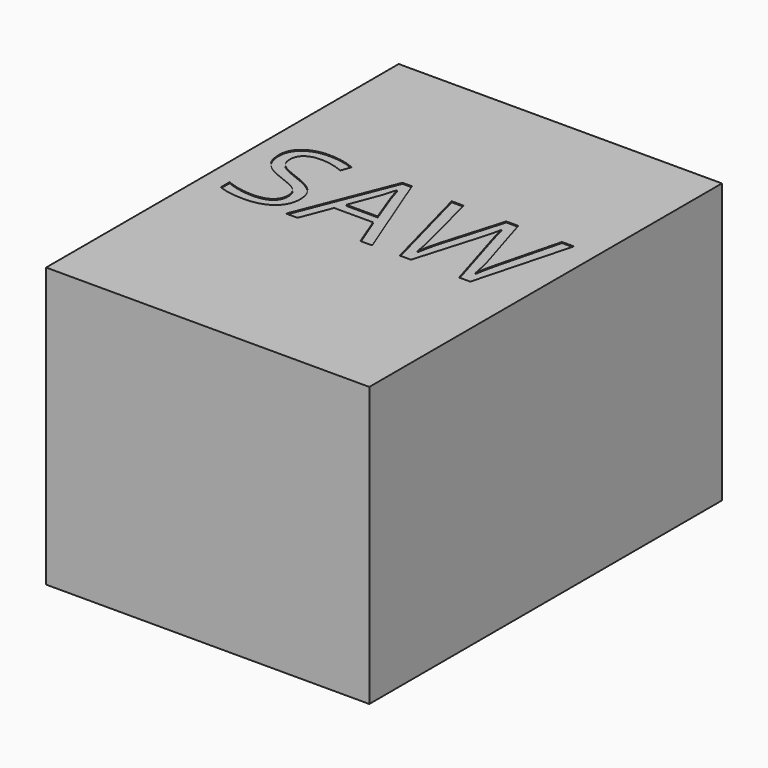
from build123d import *

# Parameters (mm, degrees)
F0_W         = 330
F0_H         = 450
F1_DEPTH     = 285
F2_TEXT_SIZE = 138.8888888889
F3_DEPTH     = 1


# Not quite as in the source:
# - Text() gives the source's letters only with a copy of the font that has no kerning and outlines rounded to 1/6400 em; it was checked with that copy


with BuildPart() as f1:
    # F0 (on Top) → F1 (new body)
    with BuildSketch(Plane.XY):
        Rectangle(F0_W, F0_H)
    extrude(amount=F1_DEPTH)

    # F2 (on face) → F3 (cut)
    with BuildSketch(Plane.XY.offset(285)):
        with Locations((-150, -32.7823804909)):
            Text('SAW', F2_TEXT_SIZE, font='Open Sans', text_align=(TextAlign.LEFT, TextAlign.BOTTOM))
    extrude(amount=-F3_DEPTH, mode=Mode.SUBTRACT)


solid = f1.part
